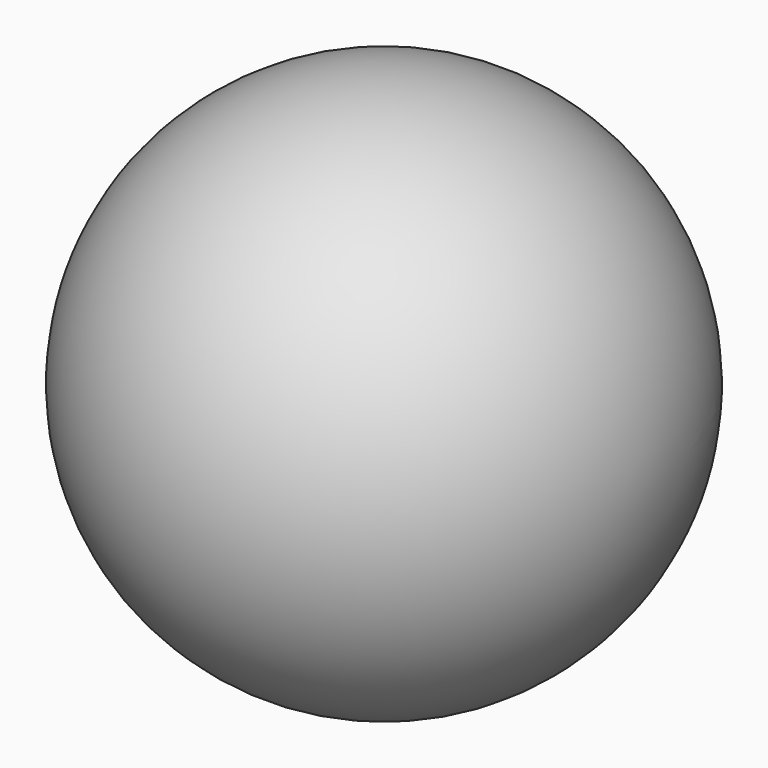
from build123d import *


with BuildPart() as f1:
    # F0 (on Top) → F1 (revolve)
    with BuildSketch(Plane.XY):
        with BuildLine():
            Line((0, 0), (26.4845338905, 0))
            ThreePointArc((26.4845338905, 0), (0, 26.4845338905), (-26.4845338905, 0))
            Line((-26.4845338905, 0), (0, 0))
        make_face()
    revolve(axis=Axis((0, 0, 0), (-1, 0, 0)))


solid = f1.part
